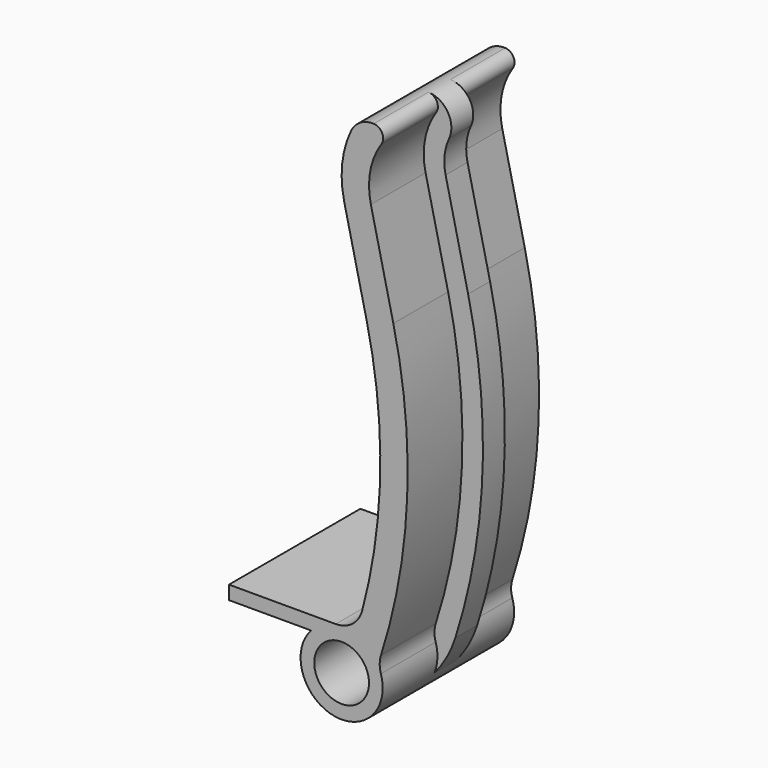
from build123d import *

# Parameters (mm, degrees)
F1_DEPTH     = 19.05
F3_W         = 4.7625
F3_H         = 6.35
F6_DEPTH     = 38.1
F8_W         = 3.175
F8_H         = 3.175
F10_R        = 6.35
F11_DEPTH    = 194
F12_R        = 2.286
F13_T1_DEPTH = 19.05
F13_T3_DEPTH = 19.05
F14_T1_DEPTH = 55.7241448987
F15_R        = 6.35


# Not quite as in the source:
# - a fillet or chamfer that OpenCascade refuses, or shapes differently, is made with other operations: its cross-section is extruded or revolved along the edge and cut away or added
# - an extrude ends at something that could not be found from the text; its depth is read off the source's solid


with BuildPart() as f1:
    # F0 (on Front) → F1 (new body, symmetric)
    with BuildSketch(Plane.XZ):
        with BuildLine():
            ThreePointArc((28.575, 0), (26.8420658771, 5.4780776161), (22.2738274294, 8.962843394))
            ThreePointArc((22.2738274294, 8.962843394), (20.6862367909, 9.3834084513), (19.05, 9.525))
            ThreePointArc((19.05, 9.525), (12.3148079092, -6.7351920908), (28.575, 0))
        make_face()
        with BuildLine():
            ThreePointArc((21.2761253017, 5.9470048042), (24.2681603878, 3.6184668255), (25.4, 0))
            ThreePointArc((25.4, 0), (13.8318396122, -3.6184668255), (21.2761253017, 5.9470048042))
        make_face(mode=Mode.SUBTRACT)
    extrude(amount=F1_DEPTH, both=True)

    # F4: sweep along a path in F0
    with BuildLine(Plane.XZ) as f4_path:
        ThreePointArc((25.4, 117.475), (19.8659933528, 107.6745739625), (19.6399690712, 96.4219079178))
        Line((19.6399690712, 96.4219079178), (24.8593203517, 73.814413767))
        ThreePointArc((24.8593203517, 73.814413767), (27.6352226284, 36.4601369227), (19.05, 0))
    # F3 (on line) → F4 (sweep)
    with BuildSketch(Plane(origin=(70.7485136742, 0, 74.2859393579), x_dir=(0.724137931, 0, -0.6896551724), z_dir=(-0.6896551724, 0, -0.724137931))):
        Polygon((-56.274137931, 19.05), (-62.624137931, 19.05), (-62.624137931, -19.05), (-56.274137931, -19.05), (-56.274137931, -3.175), (-56.274137931, 3.175), align=None)
        with Locations((-53.892887931, 0)):
            Rectangle(F3_W, F3_H)
    sweep(path=f4_path.line)

    # F5 (on face) → F6 (cut, through all)
    with BuildSketch(Plane.XZ.offset(19.05)):
        with BuildLine():
            ThreePointArc((21.2151434119, 111.3462784605), (28.6013225616, 114.0273576638), (31.2824017648, 106.6411785141))
            ThreePointArc((31.2824017648, 106.6411785141), (33.8815819119, 110.2445976054), (37.6208515055, 112.6442287212))
            Line((37.6208515055, 112.6442287212), (29.1868111498, 120.6766481076))
            ThreePointArc((29.1868111498, 120.6766481076), (24.5677298599, 116.5524963006), (21.2151434119, 111.3462784605))
        make_face()
    extrude(amount=-F6_DEPTH, mode=Mode.SUBTRACT)

    # F8 (on line) → F9 (join, up to the next surface of F1)
    with BuildSketch(Plane(origin=(-7.081156576, 0, 0), x_dir=(0, -1, 0), z_dir=(-1, 0, 0))):
        Polygon((19.05, 9.525), (-19.05, 9.525), (-19.05, 6.35), (-1.5875, 6.35), (1.5875, 6.35), (19.05, 6.35), align=None)
        with Locations((0, 4.7625)):
            Rectangle(F8_W, F8_H)
    extrude(until=Until.NEXT, dir=(1, 0, 0))

    # F10 (on face) → F11 (cut, through all)
    with BuildSketch(Plane.XZ.offset(19.05)):
        with Locations((19.05, 0)):
            Circle(F10_R)
    extrude(amount=-F11_DEPTH, mode=Mode.SUBTRACT)

    # F12
    f12_edges = [f1.edges().sort_by_distance(p)[0] for p in [
        (29.997472, -11.1125, 113.094846),
        (29.997472, 11.1125, 113.094846),
    ]]
    fillet(f12_edges, radius=F12_R)

    # F13: fillet of radius 6.35 on 1 edges, made by hand

    # F13_s2 → F13_t1 (join)
    with BuildSketch(Plane.XZ.offset(-19.05)):
        with BuildLine():
            ThreePointArc((23.8130222807, 14.2302123328), (21.5448448234, 10.8368008333), (17.6797382069, 9.525))
            Line((17.6797382069, 9.525), (17.6797382069, 8.89))
            ThreePointArc((17.6797382069, 8.89), (19.05, 8.89), (22.0589056007, 8.3653205011))
            Line((22.0589056007, 8.3653205011), (22.8792169958, 8.7711966544))
            ThreePointArc((22.8792169958, 8.7711966544), (23.68228697, 11.4098439061), (24.4263506881, 14.0657335661))
            Line((24.4263506881, 14.0657335661), (23.8130222807, 14.2302123328))
        make_face()
    extrude(amount=F13_T1_DEPTH)

    # F13_s4 → F13_t3 (join)
    with BuildSketch(Plane.XZ):
        with BuildLine():
            ThreePointArc((23.8130222807, 14.2302123328), (21.5448448234, 10.8368008333), (17.6797382069, 9.525))
            Line((17.6797382069, 9.525), (17.6797382069, 8.89))
            ThreePointArc((17.6797382069, 8.89), (19.05, 8.89), (22.0589056007, 8.3653205011))
            Line((22.0589056007, 8.3653205011), (22.8792169958, 8.7711966544))
            ThreePointArc((22.8792169958, 8.7711966544), (23.68228697, 11.4098439061), (24.4263506881, 14.0657335661))
            Line((24.4263506881, 14.0657335661), (23.8130222807, 14.2302123328))
        make_face()
    extrude(amount=F13_T3_DEPTH)

    # F14: fillet of radius 25.4 on 1 edges, made by hand

    # F14_s2 → F14_t1 (cut)
    with BuildSketch(Plane.XZ.offset(-27.8620724494)):
        with BuildLine():
            ThreePointArc((32.7132170359, 5.1228403953), (30.7267768935, 0.5385983152), (27.8814262147, -3.5681278023))
            Line((27.8814262147, -3.5681278023), (29.3533305839, -4.1628157693))
            ThreePointArc((29.3533305839, -4.1628157693), (31.1186935714, 0.4491043519), (32.7132170359, 5.1228403953))
        make_face()
    extrude(amount=F14_T1_DEPTH, mode=Mode.SUBTRACT)

    # F15
    f15_edges = [f1.edges().sort_by_distance(p)[0] for p in [
        (27.473994, -11.1125, 4.445441),
        (27.473994, 11.1125, 4.445441),
    ]]
    fillet(f15_edges, radius=F15_R)


solid = f1.part
